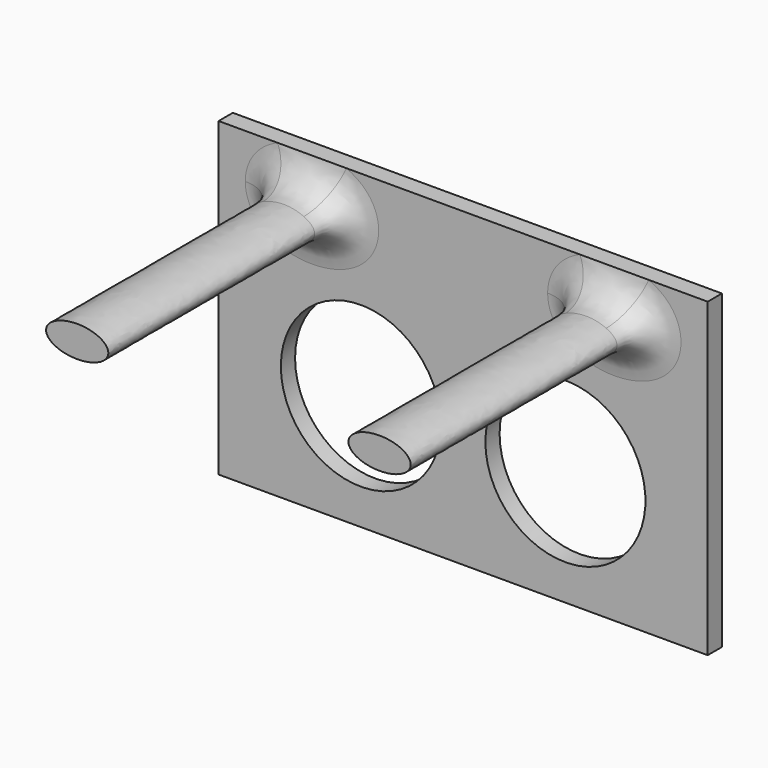
from build123d import *

# Parameters (mm, degrees)
F0_W     = 55
F0_H     = 35
F1_DEPTH = 2
F2_D     = 18
F4_DEPTH = 35
F5_R     = 4


with BuildPart() as f1:
    # F0 (on Front) → F1 (new body)
    with BuildSketch(Plane.XZ):
        with Locations((-27.5, -17.5)):
            Rectangle(F0_W, F0_H)
    extrude(amount=F1_DEPTH)

    # F2 (through all)
    with Locations(Plane(origin=(0, 0, 0), x_dir=(1, 0, 0), z_dir=(0, 1, 0))):
        with Locations((-16, 22), (-39, 22)):
            Hole(F2_D / 2)

    # F3 (on face) → F4 (join)
    with BuildSketch(Plane.XZ):
        with BuildLine():
            add(Edge.make_bspline(
                [(-14, -5), (-14, -8.0310889132), (-8.75, -6.5155444566), (-3.5, -5), (-8.75, -3.4844555434), (-14, -1.9689110868), (-14, -5)],
                knots=[0, 0, 0, 2.0943951024, 2.0943951024, 4.1887902048, 4.1887902048, 6.2831853072, 6.2831853072, 6.2831853072], degree=2, weights=[1, 0.5, 1, 0.5, 1, 0.5, 1]))
        make_face()
        with BuildLine():
            add(Edge.make_bspline(
                [(-48, -5), (-48, -8.0310889132), (-42.75, -6.5155444566), (-37.5, -5), (-42.75, -3.4844555434), (-48, -1.9689110868), (-48, -5)],
                knots=[0, 0, 0, 2.0943951024, 2.0943951024, 4.1887902048, 4.1887902048, 6.2831853072, 6.2831853072, 6.2831853072], degree=2, weights=[1, 0.5, 1, 0.5, 1, 0.5, 1]))
        make_face()
    extrude(amount=F4_DEPTH)

    # F5
    f5_edges = [f1.edges().sort_by_distance(p)[0] for p in [
        (-41, -2, -5),
        (-7, -2, -5),
    ]]
    fillet(f5_edges, radius=F5_R)


solid = f1.part
